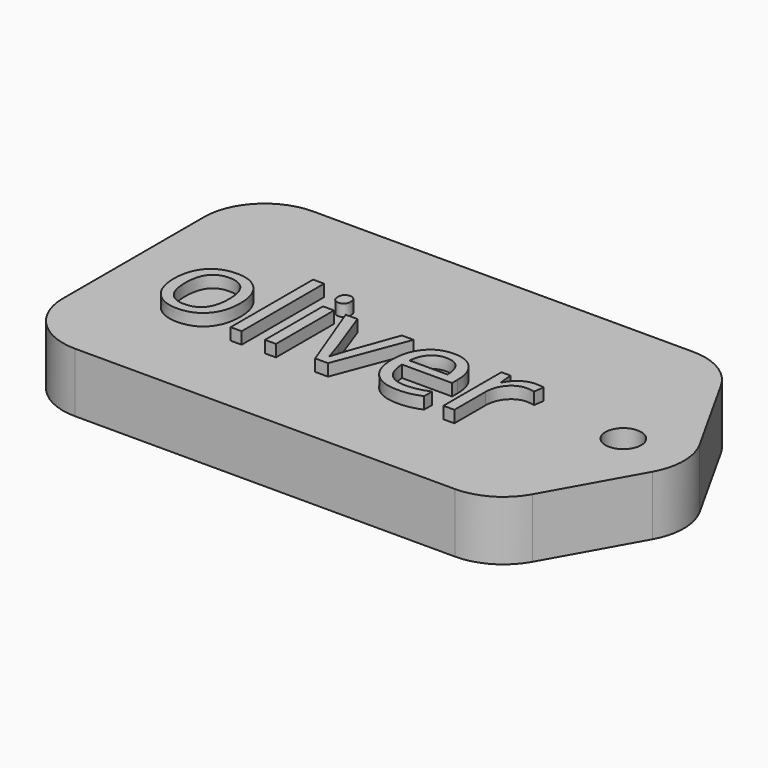
from build123d import *

# Parameters (mm, degrees)
F1_DEPTH     = 5
F2_R         = 5.08
F4_D         = 3
F5_R         = 5.08
F6_R         = 5.08
F7_R         = 5.08
F8_TEXT_SIZE = 11.4027794275
F9_DEPTH     = 1


# Not quite as in the source:
# - Text() gives the source's letters only with a copy of the font that has no kerning and outlines rounded to 1/6400 em; it was checked with that copy


with BuildPart() as f1:
    # F0 (on Top) → F1 (new body)
    with BuildSketch(Plane.XY):
        Polygon((-20, 12.5), (-20, -12.5), (20, -12.5), (26.9856210798, 0), (20, 12.5), align=None)
    extrude(amount=F1_DEPTH)

    # F2
    f2_edges = [f1.edges().sort_by_distance(p)[0] for p in [
        (26.985621, 0, 2.5),
    ]]
    fillet(f2_edges, radius=F2_R)

    # F4 (through all)
    with Locations(Plane.XY.offset(5)):
        with Locations((21.1661646207, 0)):
            Hole(F4_D / 2)

    # F5
    f5_edges = [f1.edges().sort_by_distance(p)[0] for p in [
        (20, 12.5, 2.5),
        (-20, 12.5, 2.5),
    ]]
    fillet(f5_edges, radius=F5_R)

    # F6
    f6_edges = [f1.edges().sort_by_distance(p)[0] for p in [
        (-20, -12.5, 2.5),
    ]]
    fillet(f6_edges, radius=F6_R)

    # F7
    f7_edges = [f1.edges().sort_by_distance(p)[0] for p in [
        (20, -12.5, 2.5),
    ]]
    fillet(f7_edges, radius=F7_R)

    # F8 (on face) → F9 (join)
    with BuildSketch(Plane.XY.offset(5)):
        with Locations((-15.522002295, -5.2318370088)):
            Text('oliver', F8_TEXT_SIZE, font='Open Sans', text_align=(TextAlign.LEFT, TextAlign.BOTTOM))
    extrude(amount=F9_DEPTH)


solid = f1.part
